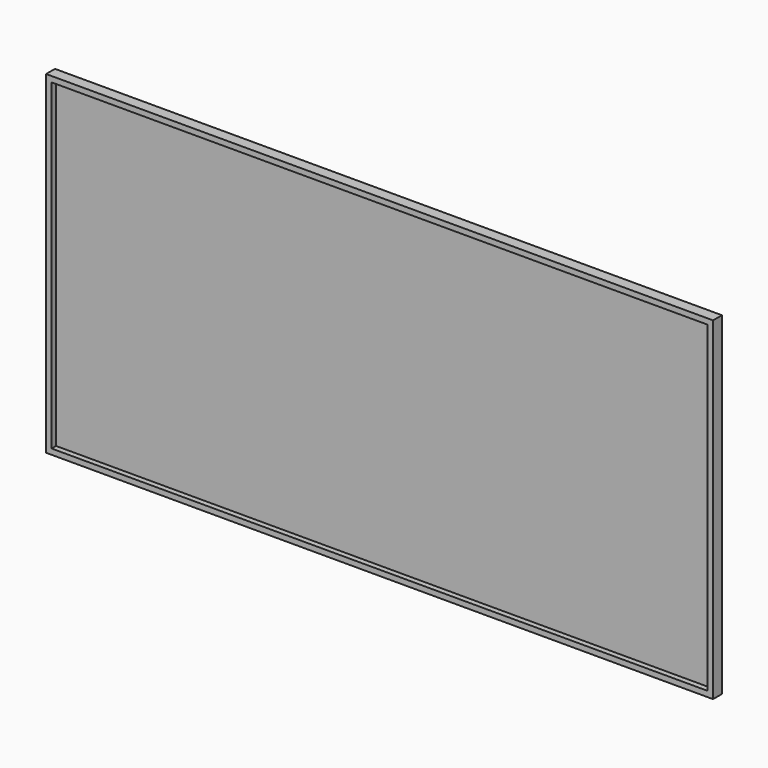
from build123d import *

# Parameters (mm, degrees)
F0_W     = 600
F0_H     = 300
F1_DEPTH = 10
F2_W     = 590.0000214577
F2_H     = 290.0000214577
F3_DEPTH = 5
F4_W     = 200
F4_H     = 150
F5_DEPTH = 30
F6_R     = 5
F7_R     = 20
F8_DEPTH = 10


with BuildPart() as f1:
    # F0 (on Front) → F1 (new body)
    with BuildSketch(Plane.XZ):
        with Locations((-100, 103.4820094705)):
            Rectangle(F0_W, F0_H)
    extrude(amount=F1_DEPTH)

    # F2 (on face) → F3 (cut)
    with BuildSketch(Plane.XZ.offset(10)):
        with Locations((-100, 103.4820094705)):
            Rectangle(F2_W, F2_H)
    extrude(amount=-F3_DEPTH, mode=Mode.SUBTRACT)

    # F4 (on face) → F5 (join)
    with BuildSketch(Plane.XZ.offset(5)):
        with Locations((-200, 125)):
            Rectangle(F4_W, F4_H)
    extrude(amount=-F5_DEPTH)

    # F6
    f6_edges = [f1.edges().sort_by_distance(p)[0] for p in [
        (-100, 0, 125),
        (-100, 12.5, 200),
        (-100, 25, 125),
        (-100, 12.5, 50),
        (-300, 0, 125),
        (-300, 12.5, 50),
        (-300, 25, 125),
        (-300, 12.5, 200),
        (-200, 0, 200),
        (-200, 0, 50),
    ]]
    fillet(f6_edges, radius=F6_R)

    # F7 (on face) → F8 (cut)
    with BuildSketch(Plane(origin=(0, 25, 0), x_dir=(-1, 0, 0), z_dir=(0, 1, 0))):
        with Locations((199.6024996042, 138.1175220013)):
            Circle(F7_R)
    extrude(amount=-F8_DEPTH, mode=Mode.SUBTRACT)


solid = f1.part
